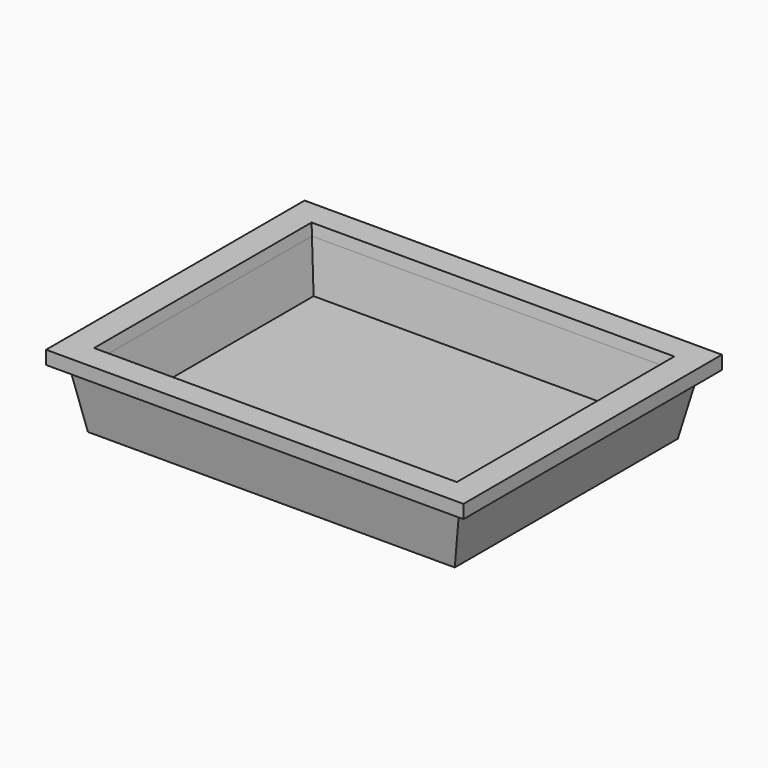
from build123d import *

# Parameters (mm, degrees)
F0_W          = 465
F0_H          = 360
F1_DEPTH      = 82
F3_DEPTH      = 238.8411541644
F3_DEPTH_BACK = 251
F5_DEPTH      = 190
F5_DEPTH_BACK = 341
F6_T          = 18
F6_T3_DEPTH   = 370.2074342574
F6_T5_DEPTH   = 471


# Not quite as in the source:
# - a shell that OpenCascade refuses in one call is made with other operations: the cavity is built on its own and cut out


with BuildPart() as f1:
    # F0 (on Top) → F1 (new body)
    with BuildSketch(Plane.XY):
        with Locations((6.3401541644, 0)):
            Rectangle(F0_W, F0_H)
    extrude(amount=-F1_DEPTH)

    # F2 (on Right) → F3 (cut, two sides)
    with BuildSketch(Plane.YZ) as f3_sk:
        Polygon((-210, -15), (-210, -112), (-150, -112), (-167.1037171287, -15), align=None)
        Polygon((210, -15), (167.1037171287, -15), (150, -112), (210, -112), align=None)
    extrude(amount=F3_DEPTH, mode=Mode.SUBTRACT)
    extrude(f3_sk.sketch, amount=-F3_DEPTH_BACK, mode=Mode.SUBTRACT)

    # F4 (on Front) → F5 (cut, two sides)
    with BuildSketch(Plane.XZ) as f5_sk:
        Polygon((-241.1598458356, -15), (-241.1598458356, -185.1384545885), (-181.1598458356, -185.1384545885), (-211.1598458356, -15), align=None)
        Polygon((253.8401541644, -15), (223.8401541644, -15), (193.8816988413, -154.3605614963), (253.8401541644, -156.5929672103), align=None)
    extrude(amount=F5_DEPTH, mode=Mode.SUBTRACT)
    extrude(f5_sk.sketch, amount=-F5_DEPTH_BACK, mode=Mode.SUBTRACT)

    # F6: shell of thickness 18, made by hand


with BuildPart() as f6_core1:
    # F6_t2: copy of F1
    add(f1.part)

    # the walls: a layer under each face that stays
    f6_faces = [f6_core1.faces().sort_by_distance(p)[0] for p in [
        (-226.1598458356, 0, -7.5),
        (6.3401541644, -180, -7.5),
        (238.8401541644, 0, -7.5),
        (223.3401541644, 168, -15),
        (6.3401541644, 161.196763275, -48.5),
        (5.0455852734, 0, -82),
        (216.6386314197, 0, -48.5),
        (6.3401541644, -161.196763275, -48.5),
        (-205.2528919819, 0, -48.5),
        (6.3401541644, 180, -7.5),
    ]]
    thicken(f6_faces, amount=-F6_T, mode=Mode.SUBTRACT)

    # F6_s4 → F6_t3 (cut)
    with BuildSketch(Plane.XZ.offset(-185.1037171287)):
        Polygon((-211.3371112312, -15.211256672), (-211.1598458356, 3), (-196.0560524744, 3), (-193.4333062814, -11.874332802), align=None)
        Polygon((224.0161338598, -15.2178305009), (223.8401541644, 3), (209.2984141185, 3), (206.2421846213, -11.2169499127), align=None)
    extrude(amount=F6_T3_DEPTH, mode=Mode.SUBTRACT)

    # F6_s6 → F6_t5 (cut)
    with BuildSketch(Plane.YZ.offset(-229.1598458356)):
        Polygon((-167.2809825243, -15.211256672), (-167.1037171287, 3), (-151.9999237675, 3), (-149.3771775745, -11.874332802), align=None)
        Polygon((167.2809825243, -15.211256672), (167.1037171287, 3), (151.9999237675, 3), (149.3771775745, -11.874332802), align=None)
    extrude(amount=F6_T5_DEPTH, mode=Mode.SUBTRACT)


with BuildPart() as f1_1:
    add(f1.part)

    # what is left inside the walls is the cavity
    f6_cavity = [f6_core1.part.solids().sort_by_distance(p)[0] for p in [
        (6.563215, -50.490314, -0.18),
    ]]
    add(f6_cavity, mode=Mode.SUBTRACT)


solid = f1_1.part
